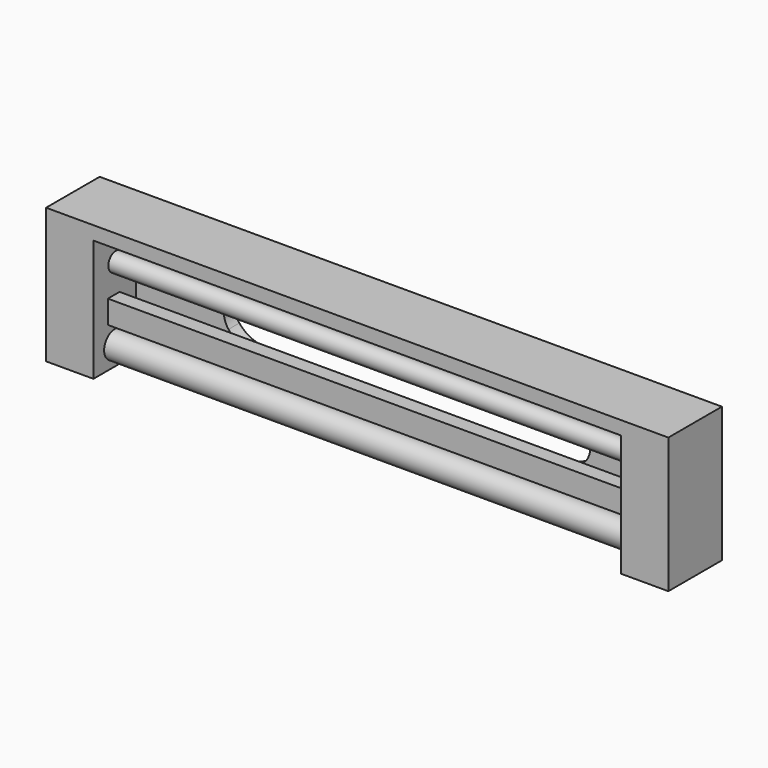
from build123d import *

# Parameters (mm, degrees)
F0_W         = 82
F0_H         = 9.9
F1_DEPTH     = 20
F2_T         = -2
F3_DEPTH     = 2
F4_DEPTH     = 5
F6_R         = 1.3971487494
F5_R         = 1.9718048452
F7_DEPTH     = 74
F8_W         = 55.0399487838
F8_H         = 7.4755754322
F9_DEPTH     = 2
F10_T1_DEPTH = 2
F11_R        = 3
F12_W        = 1.8215961754
F12_H        = 3.4220837988
F13_DEPTH    = 1
F14_T4_DEPTH = 3.4220837988
F14_T9_DEPTH = 3.4220837988
F15_R        = 0.7
F16_W        = 0.433061509
F16_H        = 3.4220837988
F16_W_2      = 1.2856977906
F16_W_3      = 0.4418755459
F17_DEPTH    = 73
F19_DEPTH    = 10
F20_DEPTH    = 5


# Not quite as in the source:
# - a fillet or chamfer that OpenCascade refuses, or shapes differently, is made with other operations: its cross-section is extruded or revolved along the edge and cut away or added
# - a feature of the source that left no trace in its solid (it failed there, or was rolled back) is left out


with BuildPart() as f1:
    # F0 (on Top) → F1 (new body)
    with BuildSketch(Plane.XY):
        with Locations((-34.3298178315, -49.909187454)):
            Rectangle(F0_W, F0_H)
    extrude(amount=F1_DEPTH)

    # F2
    f2_openings = [f1.faces().sort_by_distance(p)[0] for p in [
        (-34.329818, -54.859187, 10),
    ]]
    offset(amount=F2_T, openings=f2_openings)

    # F3 (cut): a face of the model
    f3_faces = [f1.faces().sort_by_distance(p)[0] for p in [
        (-34.3298178315, -50.909187454, 2),
    ]]
    extrude(f3_faces, amount=-F3_DEPTH, mode=Mode.SUBTRACT)

    # F4 (add): a face of the model
    f4_faces = [f1.faces().sort_by_distance(p)[0] for p in [
        (4.6701821685, -50.909187454, 9),
    ]]
    extrude(f4_faces, amount=F4_DEPTH)

    # F6 (on face) + F5 (on face) → F7 (join)
    with BuildSketch(Plane(origin=(-0.3298178315, 0, 0), x_dir=(0, -1, 0), z_dir=(-1, 0, 0))):
        with Locations((50.704728812, 13.591603376)):
            Circle(F6_R)
    with BuildSketch(Plane(origin=(-0.3298178315, 0, 0), x_dir=(0, -1, 0), z_dir=(-1, 0, 0))):
        with Locations((50.909187454, 2.9176021926)):
            Circle(F5_R)
    extrude(amount=F7_DEPTH)

    # F8 (on face) → F9 (cut)
    with BuildSketch(Plane.XZ.offset(46.959187454)):
        with Locations((-38.2777568884, 9.5675773919)):
            Rectangle(F8_W, F8_H)
    extrude(amount=-F9_DEPTH, mode=Mode.SUBTRACT)

    # F10: fillet of radius 5 on 4 edges, made by hand

    # F10_s2 → F10_t1 (join)
    with BuildSketch(Plane.XZ.offset(44.959187454)):
        with BuildLine():
            ThreePointArc((-15.7577824965, 5.8297896758), (-12.2222485906, 7.2942557698), (-10.7577824965, 10.8297896758))
            Line((-10.7577824965, 10.8297896758), (-10.7577824965, 5.8297896758))
            Line((-10.7577824965, 5.8297896758), (-15.7577824965, 5.8297896758))
        make_face()
        with BuildLine():
            ThreePointArc((-65.7977312803, 10.8297896758), (-64.3332651863, 7.2942557698), (-60.7977312803, 5.8297896758))
            Line((-60.7977312803, 5.8297896758), (-65.7977312803, 5.8297896758))
            Line((-65.7977312803, 5.8297896758), (-65.7977312803, 10.8297896758))
        make_face()
        with BuildLine():
            ThreePointArc((-60.7977312803, 13.305365108), (-64.3332651863, 11.8408990139), (-65.7977312803, 8.305365108))
            Line((-65.7977312803, 8.305365108), (-65.7977312803, 13.305365108))
            Line((-65.7977312803, 13.305365108), (-60.7977312803, 13.305365108))
        make_face()
        with BuildLine():
            ThreePointArc((-15.7577824965, 13.305365108), (-12.2222485906, 11.8408990139), (-10.7577824965, 8.305365108))
            Line((-10.7577824965, 8.305365108), (-10.7577824965, 13.305365108))
            Line((-10.7577824965, 13.305365108), (-15.7577824965, 13.305365108))
        make_face()
    extrude(amount=F10_T1_DEPTH)

    # F11
    f11_edges = [f1.edges().sort_by_distance(p)[0] for p in [
        (-10.919723, -45.959187, 9.567577),
        (-65.635791, -45.959187, 9.567577),
    ]]
    fillet(f11_edges, radius=F11_R)

    # F12 (on face) → F13 (join)
    with BuildSketch(Plane(origin=(-0.3298178315, 0, 0), x_dir=(0, -1, 0), z_dir=(-1, 0, 0))):
        with Locations((51.1129107326, 7.6496207621)):
            Rectangle(F12_W, F12_H)
    extrude(amount=F13_DEPTH)

    # F14: fillet of radius 2 on 2 edges, made by hand


with BuildPart() as f14_tool2:
    # F14_s3 → F14_t4 (new body)
    with BuildSketch(Plane.XY.offset(5.9385788627)):
        with BuildLine():
            ThreePointArc((0.6701821685, -52.0237088203), (-0.7440313939, -51.4379223827), (-1.3298178315, -50.0237088203))
            Line((-1.3298178315, -50.0237088203), (-1.3698178315, -50.0237088203))
            Line((-1.3698178315, -50.0237088203), (-1.3698178315, -52.0637088203))
            Line((-1.3698178315, -52.0637088203), (0.6701821685, -52.0637088203))
            Line((0.6701821685, -52.0637088203), (0.6701821685, -52.0237088203))
        make_face()
    extrude(amount=F14_T4_DEPTH)

    split(bisect_by=Plane.YZ.offset(-0.3298178315), keep=Keep.BOTTOM)


with BuildPart() as f1_1:
    add(f1.part)

    # F14_t1: cut F14_tool2
    add(f14_tool2.part, mode=Mode.SUBTRACT)


with BuildPart() as f14_tool7:
    # F14_s8 → F14_t9 (new body)
    with BuildSketch(Plane.XY.offset(9.3606626615)):
        with BuildLine():
            ThreePointArc((0.6701821685, -50.2021126449), (-0.7440313939, -50.7878990825), (-1.3298178315, -52.2021126449))
            Line((-1.3298178315, -52.2021126449), (-1.3698178315, -52.2021126449))
            Line((-1.3698178315, -52.2021126449), (-1.3698178315, -50.1621126449))
            Line((-1.3698178315, -50.1621126449), (0.6701821685, -50.1621126449))
            Line((0.6701821685, -50.1621126449), (0.6701821685, -50.2021126449))
        make_face()
    extrude(amount=-F14_T9_DEPTH)

    split(bisect_by=Plane.YZ.offset(-0.3298178315), keep=Keep.BOTTOM)


with BuildPart() as f1_2:
    add(f1_1.part)

    # F14_t6: cut F14_tool7
    add(f14_tool7.part, mode=Mode.SUBTRACT)

    # F15
    f15_edges = [f1_2.edges().sort_by_distance(p)[0] for p in [
        (-1.007208, -51.112911, 7.649621),
    ]]
    fillet(f15_edges, radius=F15_R)

    # F16 (on face) → F17 (join)
    with BuildSketch(Plane(origin=(-0.3298178315, 0, 0), x_dir=(0, -1, 0), z_dir=(-1, 0, 0))):
        with Locations((50.2535310828, 7.6496207621)):
            Rectangle(F16_W, F16_H)
        with Locations((51.1129107326, 7.6496207621)):
            Rectangle(F16_W_2, F16_H)
        with Locations((51.9766974008, 7.6496207621)):
            Rectangle(F16_W_3, F16_H)
    extrude(amount=F17_DEPTH)

    # F19 (add): a face of the model
    f19_faces = [f1_2.faces().sort_by_distance(p)[0] for p in [
        (-75.3298178315, -49.909187454, 10),
    ]]
    extrude(f19_faces, amount=F19_DEPTH)

    # F20 (cut): a face of the model
    f20_faces = [f1_2.faces().sort_by_distance(p)[0] for p in [
        (-73.3298178315, -50.9067397847, 9.4818900009),
    ]]
    extrude(f20_faces, amount=-F20_DEPTH, mode=Mode.SUBTRACT)


solid = f1_2.part
